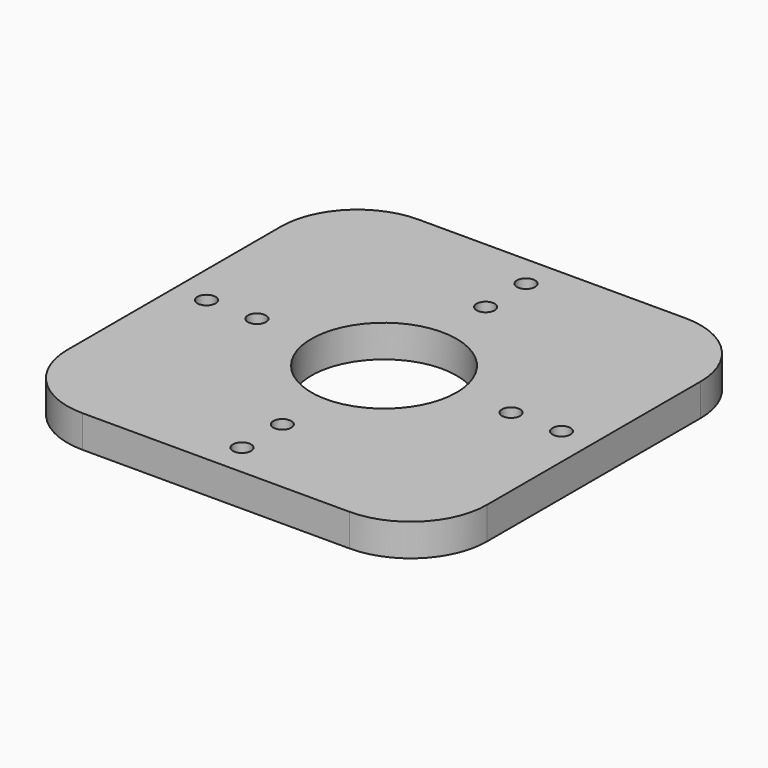
from build123d import *

# Parameters (mm, degrees)
F0_W     = 82.55
F0_H     = 82.55
F0_R     = 1.778
F0_R_2   = 14.2875
F1_DEPTH = 6.35
F2_R     = 15


# Not quite as in the source:
# - a length typed as a fraction of an inch, garbled in the dataset ("3 / 203.2 mm" for 3/8 in), is restored


with BuildPart() as f1:
    # F0 (on Top) → F1 (new body)
    with BuildSketch(Plane.XY):
        Rectangle(F0_W, F0_H)
        with Locations((0, -34.925)):
            Circle(F0_R, mode=Mode.SUBTRACT)
        with Locations((0, -25)):
            Circle(F0_R, mode=Mode.SUBTRACT)
        with Locations((-34.925, 0)):
            Circle(F0_R, mode=Mode.SUBTRACT)
        with Locations((-25, 0)):
            Circle(F0_R, mode=Mode.SUBTRACT)
        Circle(F0_R_2, mode=Mode.SUBTRACT)
        with Locations((25, 0)):
            Circle(F0_R, mode=Mode.SUBTRACT)
        with Locations((34.925, 0)):
            Circle(F0_R, mode=Mode.SUBTRACT)
        with Locations((0, 25)):
            Circle(F0_R, mode=Mode.SUBTRACT)
        with Locations((0, 34.925)):
            Circle(F0_R, mode=Mode.SUBTRACT)
    extrude(amount=F1_DEPTH)

    # F2
    f2_edges = [f1.edges().sort_by_distance(p)[0] for p in [
        (-41.275, 41.275, 3.175),
        (-41.275, -41.275, 3.175),
        (41.275, 41.275, 3.175),
        (41.275, -41.275, 3.175),
    ]]
    fillet(f2_edges, radius=F2_R)


solid = f1.part
